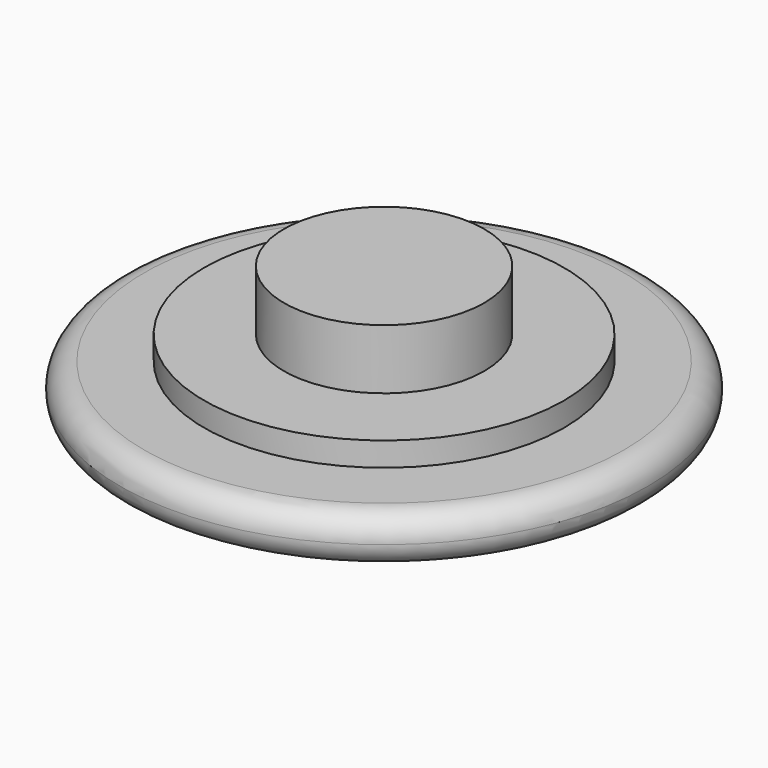
from build123d import *

# Parameters (mm, degrees)
F0_R         = 11
F0_R_2       = 7.5
F1_DEPTH     = 2
F0_R_3       = 4.175
F2_DEPTH     = 3
F3_DEPTH     = 5.5
F4_R         = 0.99999
F5_TEXT_SIZE = 10.4130016005
F6_DEPTH     = 1


# Not quite as in the source:
# - a fillet or chamfer is up to 0.001 mm smaller than in the source, because OpenCascade refuses the exact size
# - Text() gives the source's letters only with a copy of the font that has no kerning and outlines rounded to 1/6400 em; it was checked with that copy


with BuildPart() as f1:
    # F0 (on Top) → F1 (new body)
    with BuildSketch(Plane.XY):
        Circle(F0_R)
        Circle(F0_R_2, mode=Mode.SUBTRACT)
    extrude(amount=F1_DEPTH)

    # F0 (on Top) → F2 (join)
    with BuildSketch(Plane.XY):
        Circle(F0_R_2)
        Circle(F0_R_3, mode=Mode.SUBTRACT)
    extrude(amount=F2_DEPTH)

    # F0 (on Top) → F3 (join)
    with BuildSketch(Plane.XY):
        Circle(F0_R_3)
    extrude(amount=F3_DEPTH)

    # F4 (radius 1 in the source; OpenCascade refuses exactly that, so slightly less here)
    f4_edges = [f1.edges().sort_by_distance(p)[0] for p in [
        (-11, 0, 2),
        (-11, 0, 0),
    ]]
    fillet(f4_edges, radius=F4_R)

    # F5 (on face) → F6 (cut)
    with BuildSketch(Plane(origin=(0, 0, 0), x_dir=(1, 0, 0), z_dir=(0, 0, -1))):
        with Locations((-9.3474228196, -3.5532642221)):
            Text('Pap', F5_TEXT_SIZE, font='Open Sans', text_align=(TextAlign.LEFT, TextAlign.BOTTOM))
    extrude(amount=-F6_DEPTH, mode=Mode.SUBTRACT)


solid = f1.part
